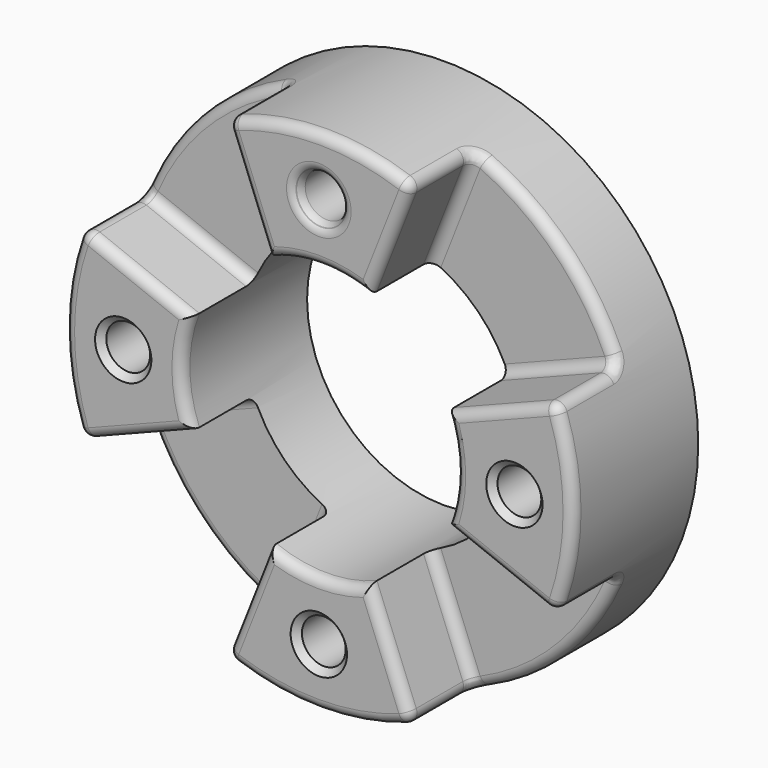
from build123d import *

# Parameters (mm, degrees)
F0_R     = 20.6375
F0_R_2   = 1.778
F0_R_3   = 11.1125
F1_DEPTH = 12.7
F2_SIZE  = 0.508
F4_DEPTH = 6.35
F6_R     = 0.8128


# Not quite as in the source:
# - a feature of the source that left no trace in its solid (it failed there, or was rolled back) is left out


with BuildPart() as f1:
    # F0 (on Front) → F1 (new body)
    with BuildSketch(Plane.XZ):
        Circle(F0_R)
        with Locations((0, -15.875)):
            Circle(F0_R_2, mode=Mode.SUBTRACT)
        with Locations((-15.875, 0)):
            Circle(F0_R_2, mode=Mode.SUBTRACT)
        Circle(F0_R_3, mode=Mode.SUBTRACT)
        with Locations((15.875, 0)):
            Circle(F0_R_2, mode=Mode.SUBTRACT)
        with Locations((0, 15.875)):
            Circle(F0_R_2, mode=Mode.SUBTRACT)
    extrude(amount=F1_DEPTH)

    # F2
    f2_edges = [f1.edges().sort_by_distance(p)[0] for p in [
        (-17.653, -12.7, 0),
        (-1.778, -12.7, 15.875),
        (14.097, -12.7, 0),
        (-1.778, -12.7, -15.875),
    ]]
    chamfer(f2_edges, length=F2_SIZE)

    # F3 (on face) → F4 (cut)
    with BuildSketch(Plane.XZ.offset(12.7)):
        with BuildLine():
            Line((10.3392652242, 4.072744882), (19.2014925592, 7.5636690665))
            ThreePointArc((19.2014925592, 7.5636690665), (14.5929161967, 14.5929161967), (7.5636690665, 19.2014925592))
            Line((7.5636690665, 19.2014925592), (4.072744882, 10.3392652242))
            ThreePointArc((4.072744882, 10.3392652242), (7.8577241059, 7.8577241059), (10.3392652242, 4.072744882))
        make_face()
        with BuildLine():
            ThreePointArc((7.5636690665, -19.2014925592), (14.5929161967, -14.5929161967), (19.2014925592, -7.5636690665))
            Line((19.2014925592, -7.5636690665), (10.3392652242, -4.072744882))
            ThreePointArc((10.3392652242, -4.072744882), (7.8577241059, -7.8577241059), (4.072744882, -10.3392652242))
            Line((4.072744882, -10.3392652242), (7.5636690665, -19.2014925592))
        make_face()
        with BuildLine():
            Line((-7.5636690665, -19.2014925592), (-4.072744882, -10.3392652242))
            ThreePointArc((-4.072744882, -10.3392652242), (-7.8577241059, -7.8577241059), (-10.3392652242, -4.072744882))
            Line((-10.3392652242, -4.072744882), (-19.2014925592, -7.5636690665))
            ThreePointArc((-19.2014925592, -7.5636690665), (-14.5929161967, -14.5929161967), (-7.5636690665, -19.2014925592))
        make_face()
        with BuildLine():
            Line((-4.072744882, 10.3392652242), (-7.5636690665, 19.2014925592))
            ThreePointArc((-7.5636690665, 19.2014925592), (-14.5929161967, 14.5929161967), (-19.2014925592, 7.5636690665))
            Line((-19.2014925592, 7.5636690665), (-10.3392652242, 4.072744882))
            ThreePointArc((-10.3392652242, 4.072744882), (-7.8577241059, 7.8577241059), (-4.072744882, 10.3392652242))
        make_face()
    extrude(amount=-F4_DEPTH, mode=Mode.SUBTRACT)

    # F6
    f6_edges = [f1.edges().sort_by_distance(p)[0] for p in [
        (-20.6375, -12.7, 0),
        (0, -12.7, 20.6375),
        (2.032, -12.446, 15.875),
        (-1.778, -12.192, 15.875),
        (-2.286, -12.7, 15.875),
        (0, -12.7, -20.6375),
        (-5.818207, -12.7, -14.770379),
        (0, -12.7, -11.1125),
        (5.818207, -12.7, -14.770379),
        (20.27532, -12.7, -3.84939),
        (19.201493, -9.525, -7.563669),
        (14.592916, -6.35, -14.592916),
        (7.563669, -9.525, -19.201493),
        (-7.563669, -9.525, -19.201493),
        (-14.592916, -6.35, -14.592916),
        (-19.201493, -9.525, -7.563669),
        (-19.201493, -9.525, 7.563669),
        (-14.592916, -6.35, 14.592916),
        (-7.563669, -9.525, 19.201493),
        (7.563669, -9.525, 19.201493),
        (14.592916, -6.35, 14.592916),
        (19.201493, -9.525, 7.563669),
        (20.27532, -12.7, 3.84939),
        (10.91748, -12.7, -2.072748),
        (-11.1125, -12.7, 0),
        (0, -12.7, 11.1125),
        (10.91748, -12.7, 2.072748),
        (-5.818207, -6.35, -14.770379),
        (5.818207, -6.35, -14.770379),
        (14.770379, -12.7, -5.818207),
        (14.770379, -12.7, 5.818207),
        (14.770379, -6.35, -5.818207),
        (-14.770379, -6.35, -5.818207),
        (-14.770379, -12.7, -5.818207),
        (-14.770379, -12.7, 5.818207),
        (-14.770379, -6.35, 5.818207),
        (-5.818207, -6.35, 14.770379),
        (-5.818207, -12.7, 14.770379),
        (5.818207, -12.7, 14.770379),
        (5.818207, -6.35, 14.770379),
        (14.770379, -6.35, 5.818207),
    ]]
    fillet(f6_edges, radius=F6_R)


solid = f1.part
